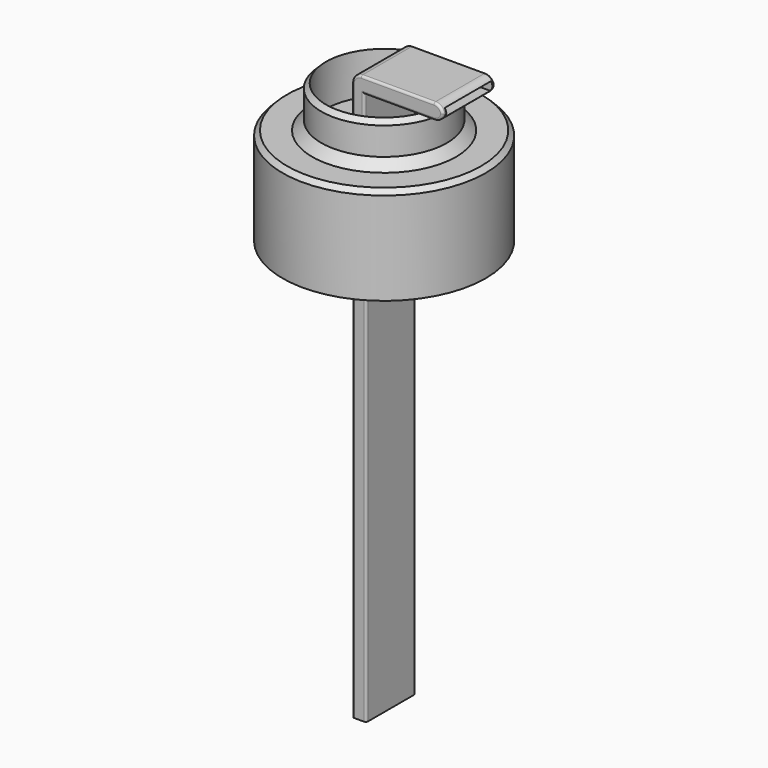
from build123d import *

# Parameters (mm, degrees)
F0_R         = 56.0284560605
F1_DEPTH     = 56.18732
F2_T         = -2.54
F3_W         = 7.7828075737
F3_H         = 34.1701302677
F4_DEPTH     = 276.60562
F6_R         = 34.5946759053
F7_DEPTH     = 25.4
F8_T         = 2.54
F8_T3_DEPTH  = 39.2501302677
F8_T5_DEPTH  = 12.8628075737
F10_SIZE     = 2.54
F11_W        = 6.7604319192
F11_H        = 35.768898204
F12_DEPTH    = 28.2828
F13_W        = 6.7604319192
F13_H        = 35.768898204
F14_DEPTH    = 6.19419
F15_W        = 35.768898204
F15_H        = 8.6004413581
F16_DEPTH    = 43.51639
F17_W        = 31.8477451801
F17_H        = 4.8072040081
F18_DEPTH    = 48.07886
F19_DEPTH    = 32.39902
F20_R        = 5.08
F21_T1_DEPTH = 61.168898204
F22_R        = 1.27


# Not quite as in the source:
# - a fillet or chamfer that OpenCascade refuses, or shapes differently, is made with other operations: its cross-section is extruded or revolved along the edge and cut away or added
# - a shell that OpenCascade refuses in one call is made with other operations: the cavity is built on its own and cut out


with BuildPart() as f1:
    # F0 (on Top) → F1 (new body)
    with BuildSketch(Plane.XY):
        Circle(F0_R)
    extrude(amount=F1_DEPTH)

    # F2
    f2_openings = [f1.faces().sort_by_distance(p)[0] for p in [
        (0, 0, 0),
    ]]
    offset(amount=F2_T, openings=f2_openings)

    # F3 (on face) → F4 (join)
    with BuildSketch(Plane(origin=(0, 0, 53.64732), x_dir=(1, 0, 0), z_dir=(0, 0, -1))):
        with Locations((0.0409056073, 0.1802544365)):
            Rectangle(F3_W, F3_H)
    extrude(amount=F4_DEPTH)

    # F5: chamfer of 5.08 on 1 edges, made by hand

    # F5_s1 → F5_t2 (revolve, cut)
    with BuildSketch(Plane.XZ):
        Polygon((58.5684560605, 0), (53.4884560605, 5.08), (53.4884560605, 0), align=None)
    revolve(axis=Axis((0, 0, 0), (0, 0, 1)), mode=Mode.SUBTRACT)

    # F6 (on face) → F7 (join)
    with BuildSketch(Plane.XY.offset(56.18732)):
        Circle(F6_R)
    extrude(amount=F7_DEPTH)

    # F8: shell of thickness 2.54, made by hand


with BuildPart() as f8_core1:
    # F8_t2: copy of F1
    add(f1.part)

    # the walls: a layer under each face that stays
    f8_faces = [f8_core1.faces().sort_by_distance(p)[0] for p in [
        (-56.0284560605, 0, 29.36366),
        (-54.7584560605, 0, 3.81),
        (-37.3523040403, -37.3523040403, 56.18732),
        (-53.4884560605, 0, 29.36366),
        (-34.5946759053, 0, 68.88732),
        (-35.658970707, -35.658970707, 53.64732),
        (3.9323093942, -0.1802544365, -84.65549),
        (0.0409056073, 16.9048106974, -84.65549),
        (-3.8504981795, -0.1802544365, -84.65549),
        (0.0409056073, -17.2653195703, -84.65549),
    ]]
    thicken(f8_faces, amount=-F8_T, mode=Mode.SUBTRACT)

    # F8_s4 → F8_t3 (cut)
    with BuildSketch(Plane.XZ.offset(-19.4448106974)):
        Polygon((3.9577093942, 53.62192), (3.9323093942, 56.18732), (1.3923093942, 56.18732), (1.3923093942, 53.64732), align=None)
        Polygon((-3.8758981795, 53.62192), (-3.8504981795, 56.18732), (-1.3104981795, 56.18732), (-1.3104981795, 53.64732), align=None)
    extrude(amount=F8_T3_DEPTH, mode=Mode.SUBTRACT)

    # F8_s6 → F8_t5 (cut)
    with BuildSketch(Plane.YZ.offset(-6.3904981795)):
        Polygon((16.9302106974, 53.62192), (16.9048106974, 56.18732), (14.3648106974, 56.18732), (14.3648106974, 53.64732), align=None)
        Polygon((-17.2907195703, 53.62192), (-17.2653195703, 56.18732), (-14.7253195703, 56.18732), (-14.7253195703, 53.64732), align=None)
    extrude(amount=F8_T5_DEPTH, mode=Mode.SUBTRACT)

    # F8_s7 → F8_t8 (revolve, cut)
    with BuildSketch(Plane.XZ):
        Polygon((34.6200759053, 56.21272), (34.5946759053, 53.64732), (32.0546759053, 53.64732), (32.0546759053, 56.18732), align=None)
    revolve(axis=Axis((0, 0, 56.18732), (0, 0, 1)), mode=Mode.SUBTRACT)

    # F8_s9 → F8_t10 (revolve, cut)
    with BuildSketch(Plane.XZ):
        Polygon((53.4630560605, 53.62192), (56.0284560605, 53.64732), (56.0284560605, 56.18732), (53.4884560605, 56.18732), align=None)
    revolve(axis=Axis((0, 0, 53.64732), (0, 0, -1)), mode=Mode.SUBTRACT)


with BuildPart() as f1_1:
    add(f1.part)

    # what is left inside the walls is the cavity
    f8_cavity = [f8_core1.part.solids().sort_by_distance(p)[0] for p in [
        (1.366909, -5.028609, -83.38549),
    ]]
    add(f8_cavity, mode=Mode.SUBTRACT)

    # F9: chamfer of 5.08 on 2 edges, made by hand

    # F9_s1 → F9_t2 (revolve)
    with BuildSketch(Plane.XZ):
        Polygon((39.6746759053, 56.18732), (34.5946759053, 61.26732), (34.5946759053, 56.18732), align=None)
    revolve(axis=Axis((0, 0, 56.18732), (0, 0, 1)))

    # F9_s3 → F9_t4 (revolve, cut)
    with BuildSketch(Plane.XZ):
        Polygon((34.5946759053, 76.50732), (29.5146759053, 81.58732), (34.5946759053, 81.58732), align=None)
    revolve(axis=Axis((0, 0, 81.58732), (0, 0, 1)), mode=Mode.SUBTRACT)

    # F10
    f10_edges = [f1_1.edges().sort_by_distance(p)[0] for p in [
        (-56.028456, 0, 56.18732),
    ]]
    chamfer(f10_edges, length=F10_SIZE)

    # F11 (on face) → F12 (join)
    with BuildSketch(Plane.XY.offset(56.18732)):
        with Locations((0.176892383, -0.2430817112)):
            Rectangle(F11_W, F11_H)
    extrude(amount=F12_DEPTH)

    # F13 (on face) → F14 (join)
    with BuildSketch(Plane.XY.offset(84.47012)):
        with Locations((0.176892383, -0.2430817112)):
            Rectangle(F13_W, F13_H)
    extrude(amount=F14_DEPTH)

    # F15 (on face) → F16 (join)
    with BuildSketch(Plane.YZ.offset(3.5571083426)):
        with Locations((-0.2430817112, 86.3640893209)):
            Rectangle(F15_W, F15_H)
    extrude(amount=F16_DEPTH)

    # F17 (on face) → F18 (cut)
    with BuildSketch(Plane.YZ.offset(47.0734983426)):
        with Locations((0.0361893326, 86.1349776387)):
            Rectangle(F17_W, F17_H)
    extrude(amount=-F18_DEPTH, mode=Mode.SUBTRACT)

    # F19 (cut): a face of the model
    f19_faces = [f1_1.faces().sort_by_distance(p)[0] for p in [
        (0.0409056074, -0.1802544364, 56.18732),
    ]]
    extrude(f19_faces, amount=-F19_DEPTH, mode=Mode.SUBTRACT)

    # F20
    f20_edges = [f1_1.edges().sort_by_distance(p)[0] for p in [
        (-3.203324, -0.243082, 90.66431),
    ]]
    fillet(f20_edges, radius=F20_R)

    # F21: fillet of radius 5.08 on 2 edges, made by hand

    # F21_s2 → F21_t1 (cut)
    with BuildSketch(Plane.XZ.offset(-30.3413673908)):
        with BuildLine():
            ThreePointArc((41.9934983426, 90.66431), (45.5856007911, 89.1764124484), (47.0734983426, 85.58431))
            Line((47.0734983426, 85.58431), (47.0734983426, 90.66431))
            Line((47.0734983426, 90.66431), (41.9934983426, 90.66431))
        make_face()
        with BuildLine():
            ThreePointArc((47.0734983426, 87.1438686419), (45.5856007911, 83.5517661934), (41.9934983426, 82.0638686419))
            Line((41.9934983426, 82.0638686419), (47.0734983426, 82.0638686419))
            Line((47.0734983426, 82.0638686419), (47.0734983426, 87.1438686419))
        make_face()
    extrude(amount=F21_T1_DEPTH, mode=Mode.SUBTRACT)

    # F22
    f22_edges = [f1_1.edges().sort_by_distance(p)[0] for p in [
        (21.935087, -18.127531, 90.66431),
        (21.935087, 17.641367, 90.66431),
        (22.775303, -18.127531, 82.063869),
        (22.775303, 17.641367, 82.063869),
        (3.557108, -18.127531, 69.125594),
        (3.557108, 17.641367, 69.125594),
        (3.932309, 16.904811, -84.65549),
        (3.932309, -17.26532, -84.65549),
        (-3.850498, 16.904811, -84.65549),
        (-3.850498, -17.26532, -84.65549),
    ]]
    fillet(f22_edges, radius=F22_R)


solid = f1_1.part
